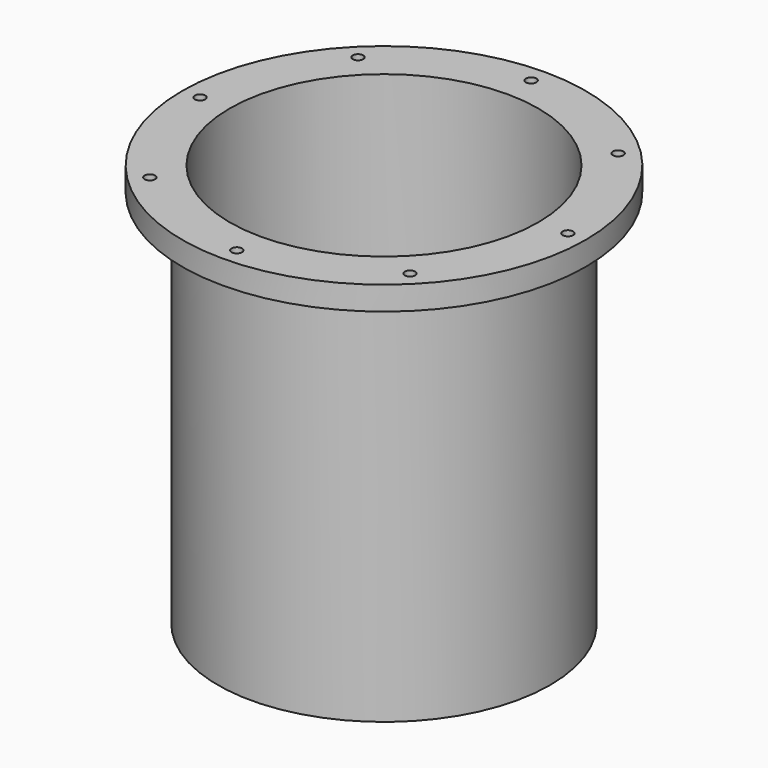
from build123d import *

# Parameters (mm, degrees)
F0_R            = 107.95
F1_DEPTH        = 12.7
F2_R            = 88.9
F3_DEPTH        = 203.2
F4_R            = 82.55
F5_DEPTH        = 203.2
F7_D            = 5.6134
F7_CSINK_D      = 10.4394
F7_CSINK_ANGLE  = 82
F7_COPIES_COUNT = 8


# Not quite as in the source:
# - a pattern or mirror of a feature is missing from the dataset's text; its kind, count and spacing are read off the source's solid


with BuildPart() as f1:
    # F0 (on Top) → F1 (new body)
    with BuildSketch(Plane.XY):
        Circle(F0_R)
    extrude(amount=-F1_DEPTH)

    # F2 (on face) → F3 (join)
    with BuildSketch(Plane(origin=(0, 0, -12.7), x_dir=(1, 0, 0), z_dir=(0, 0, -1))):
        Circle(F2_R)
    extrude(amount=F3_DEPTH)

    # F4 (on face) → F5 (cut)
    with BuildSketch(Plane.XY):
        Circle(F4_R)
    extrude(amount=-F5_DEPTH, mode=Mode.SUBTRACT)

    # F7 (through all)
    with Locations(Plane(origin=(0, 0, -12.7), x_dir=(1, 0, 0), z_dir=(0, 0, -1))):
        with Locations((0, -98.425)):
            f7 = CounterSinkHole(F7_D / 2, F7_CSINK_D / 2, counter_sink_angle=F7_CSINK_ANGLE)

    # F7_copies: F7 ×8 about axis
    f7_copies_axis = Axis((0, 0, 0), (0, 0, 1))
    for i in range(1, F7_COPIES_COUNT):
        add(f7.rotate(f7_copies_axis, i * 360 / F7_COPIES_COUNT), mode=Mode.SUBTRACT)


solid = f1.part
